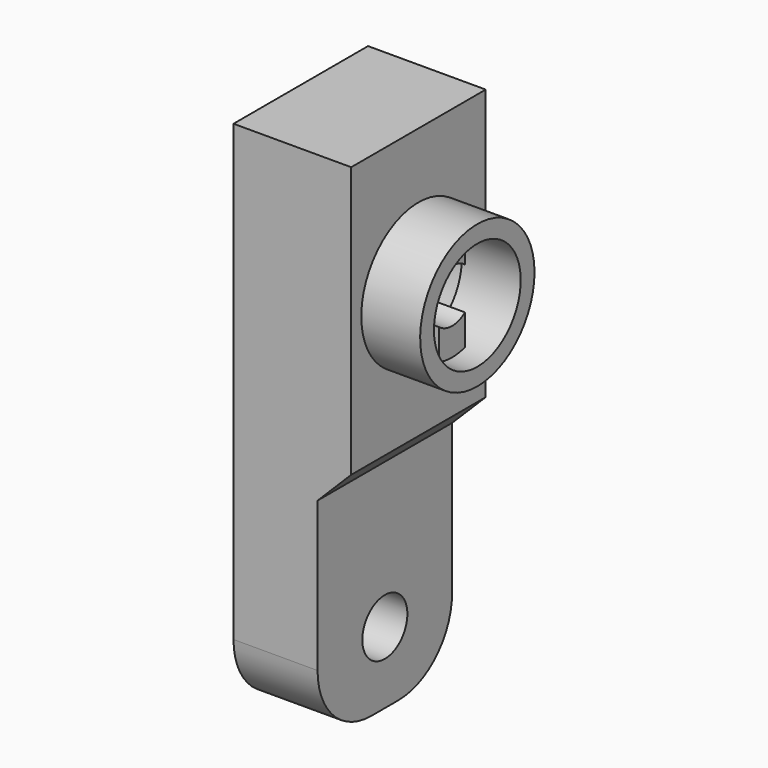
from build123d import *

# Parameters (mm, degrees)
F0_W      = 20
F0_H      = 62
F1_DEPTH  = 14
F2_R      = 8.5
F3_DEPTH  = 7
F5_D      = 12.9
F5_DEPTH  = 7
F5_TIP    = 3.8755509927
F6_W      = 3.8587664786
F6_H      = 16.5562349188
F7_DEPTH  = 11.59683
F9_D      = 6.3
F10_R     = 6.45
F11_DEPTH = 3
F12_R     = 8
F13_R     = 8
F14_W     = 4
F14_H     = 37.0940975845
F15_DEPTH = 25
F17_D     = 6.7
F18_SIZE  = 3.99999


# Not quite as in the source:
# - a fillet or chamfer is up to 0.001 mm smaller than in the source, because OpenCascade refuses the exact size


with BuildPart() as f1:
    # F0 (on Right) → F1 (new body)
    with BuildSketch(Plane.YZ):
        with Locations((-10, -31)):
            Rectangle(F0_W, F0_H)
    extrude(amount=F1_DEPTH)

    # F2 (on face) → F3 (join)
    with BuildSketch(Plane.YZ.offset(14)):
        with Locations((-10, -16.2361655384)):
            Circle(F2_R)
    extrude(amount=F3_DEPTH)

    # F5
    with Locations(Plane.YZ.offset(21)):
        with Locations((-10, -16.2361655384)):
            Hole(F5_D / 2, depth=F5_DEPTH)
            with Locations((0, 0, -(F5_DEPTH + F5_TIP / 2))):  # 118° drill point
                Cone(0, F5_D / 2, F5_TIP, mode=Mode.SUBTRACT)

    # F6 (on face) → F7 (join)
    with BuildSketch(Plane.YZ.offset(21)):
        with Locations((-10.015449224, -16.2397662935)):
            Rectangle(F6_W, F6_H)
    extrude(amount=-F7_DEPTH)

    # F9 (through all)
    with Locations(Plane.YZ.offset(21)):
        with Locations((-10, -16.2361655384)):
            Hole(F9_D / 2)

    # F10 (on face) → F11 (cut)
    with BuildSketch(Plane.YZ.offset(21)):
        with Locations((-10, -16.2361655384)):
            Circle(F10_R)
    extrude(amount=-F11_DEPTH, mode=Mode.SUBTRACT)

    # F12
    f12_edges = [f1.edges().sort_by_distance(p)[0] for p in [
        (7, 0, -62),
    ]]
    fillet(f12_edges, radius=F12_R)

    # F13
    f13_edges = [f1.edges().sort_by_distance(p)[0] for p in [
        (7, -20, -62),
    ]]
    fillet(f13_edges, radius=F13_R)

    # F14 (on face) → F15 (cut)
    with BuildSketch(Plane.XZ.offset(20)):
        with Locations((12, -50.7526341826)):
            Rectangle(F14_W, F14_H)
    extrude(amount=-F15_DEPTH, mode=Mode.SUBTRACT)

    # F17 (through all)
    with Locations(Plane(origin=(0, 0, 0), x_dir=(0, -1, 0), z_dir=(-1, 0, 0))):
        with Locations((10, -53.5)):
            Hole(F17_D / 2)

    # F18 (size 4 in the source; OpenCascade refuses exactly that, so slightly less here)
    f18_edges = [f1.edges().sort_by_distance(p)[0] for p in [
        (10, -10, -32.205585),
    ]]
    chamfer(f18_edges, length=F18_SIZE)


solid = f1.part
